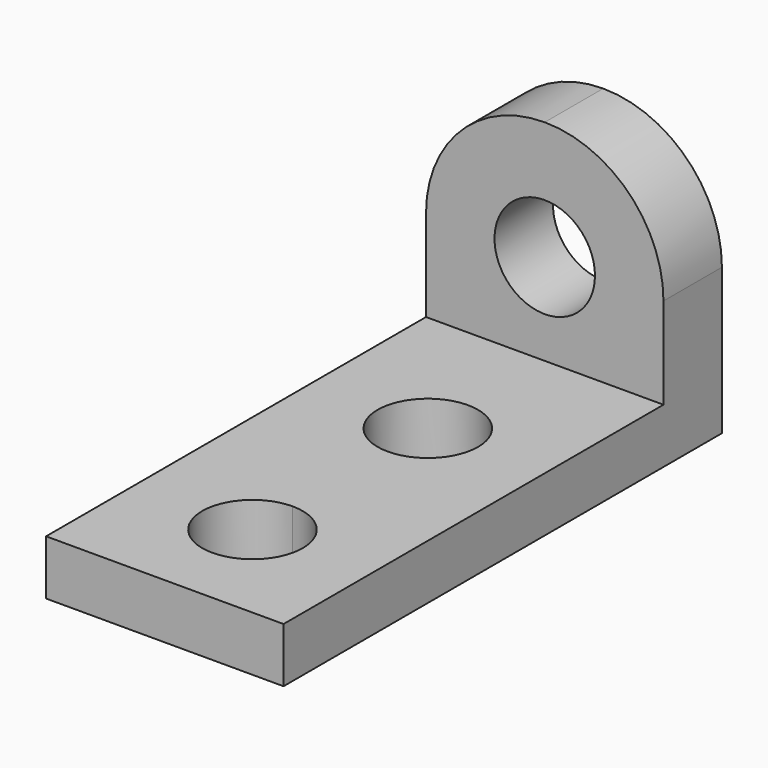
from build123d import *

# Parameters (mm, degrees)
F0_W     = 82.55
F0_H     = 190.5
F1_DEPTH = 19.05
F2_W     = 82.55
F2_H     = 25.4
F3_DEPTH = 73.025
F4_R     = 41.27499
F5_R     = 17.4625
F6_DEPTH = 25.4
F8_DEPTH = 25.4


# Not quite as in the source:
# - a fillet or chamfer is up to 0.001 mm smaller than in the source, because OpenCascade refuses the exact size


with BuildPart() as f1:
    # F0 (on Top) → F1 (new body)
    with BuildSketch(Plane.XY):
        with Locations((41.275, 95.25)):
            Rectangle(F0_W, F0_H)
    extrude(amount=F1_DEPTH)

    # F2 (on face) → F3 (join)
    with BuildSketch(Plane.XY.offset(19.05)):
        with Locations((41.275, 177.8)):
            Rectangle(F2_W, F2_H)
    extrude(amount=F3_DEPTH)

    # F4 (radius 41.275 in the source; OpenCascade refuses exactly that, so slightly less here)
    f4_edges = [f1.edges().sort_by_distance(p)[0] for p in [
        (0, 177.8, 92.075),
        (82.55, 177.8, 92.075),
    ]]
    fillet(f4_edges, radius=F4_R)

    # F5 (on face) → F6 (cut)
    with BuildSketch(Plane.XZ.offset(-165.1)):
        with Locations((41.275, 50.8)):
            Circle(F5_R)
    extrude(amount=-F6_DEPTH, mode=Mode.SUBTRACT)

    # F7 (on face) → F8 (cut)
    with BuildSketch(Plane.XY.offset(19.05)):
        with BuildLine():
            ThreePointArc((58.7375, 114.3), (28.9271478335, 126.6478521665), (41.275, 96.8375))
            ThreePointArc((41.275, 96.8375), (53.6228521665, 101.9521478335), (58.7375, 114.3))
        make_face()
        with BuildLine():
            Line((41.275, 38.1), (41.275, 20.6375))
            ThreePointArc((41.275, 20.6375), (53.6228521665, 25.7521478335), (58.7375, 38.1))
            ThreePointArc((58.7375, 38.1), (53.6228521665, 50.4478521665), (41.275, 55.5625))
            Line((41.275, 55.5625), (41.275, 38.1))
        make_face()
        with BuildLine():
            ThreePointArc((41.275, 55.5625), (23.8125, 38.1), (41.275, 20.6375))
            Line((41.275, 20.6375), (41.275, 38.1))
            Line((41.275, 38.1), (41.275, 55.5625))
        make_face()
    extrude(amount=-F8_DEPTH, mode=Mode.SUBTRACT)


solid = f1.part
